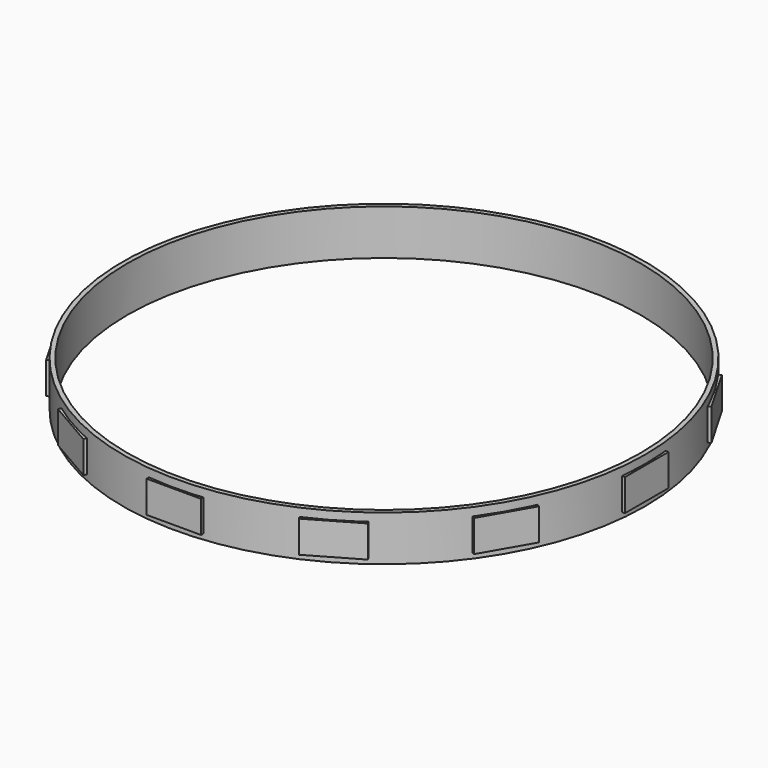
from build123d import *

# Parameters (mm, degrees)
F0_R     = 287.5
F0_R_2   = 282.5
F1_DEPTH = 50
F5_W     = 60
F5_H     = 35
F6_DEPTH = 2
F7_COUNT = 12


# Not quite as in the source:
# - the program builds the solid bodies; features that only make, move or delete a surface that nothing else refers to are left out


with BuildPart() as f1:
    # F0 (on Top) → F1 (new body)
    with BuildSketch(Plane.XY):
        Circle(F0_R)
        Circle(F0_R_2, mode=Mode.SUBTRACT)
    extrude(amount=F1_DEPTH)


with BuildPart() as f6:
    # F5 (on offset) → F6 (new body, symmetric)
    with BuildSketch(Plane.XZ.offset(287.2)):
        with Locations((0, 23.5)):
            Rectangle(F5_W, F5_H)
    extrude(amount=F6_DEPTH, both=True)


with BuildPart() as f7_1:
    # F7: instance of F6
    add(f6.part.rotate(Axis((0, 0, 0), (0, 0, -1)), 1 * 360 / F7_COUNT))


with BuildPart() as f7_2:
    # F7: instance of F6
    add(f6.part.rotate(Axis((0, 0, 0), (0, 0, -1)), 2 * 360 / F7_COUNT))


with BuildPart() as f7_3:
    # F7: instance of F6
    add(f6.part.rotate(Axis((0, 0, 0), (0, 0, -1)), 3 * 360 / F7_COUNT))


with BuildPart() as f7_4:
    # F7: instance of F6
    add(f6.part.rotate(Axis((0, 0, 0), (0, 0, -1)), 4 * 360 / F7_COUNT))


with BuildPart() as f7_5:
    # F7: instance of F6
    add(f6.part.rotate(Axis((0, 0, 0), (0, 0, -1)), 5 * 360 / F7_COUNT))


with BuildPart() as f7_6:
    # F7: instance of F6
    add(f6.part.rotate(Axis((0, 0, 0), (0, 0, -1)), 6 * 360 / F7_COUNT))


with BuildPart() as f7_7:
    # F7: instance of F6
    add(f6.part.rotate(Axis((0, 0, 0), (0, 0, -1)), 7 * 360 / F7_COUNT))


with BuildPart() as f7_8:
    # F7: instance of F6
    add(f6.part.rotate(Axis((0, 0, 0), (0, 0, -1)), 8 * 360 / F7_COUNT))


with BuildPart() as f7_9:
    # F7: instance of F6
    add(f6.part.rotate(Axis((0, 0, 0), (0, 0, -1)), 9 * 360 / F7_COUNT))


with BuildPart() as f7_10:
    # F7: instance of F6
    add(f6.part.rotate(Axis((0, 0, 0), (0, 0, -1)), 10 * 360 / F7_COUNT))


with BuildPart() as f7_11:
    # F7: instance of F6
    add(f6.part.rotate(Axis((0, 0, 0), (0, 0, -1)), 11 * 360 / F7_COUNT))


solid = Compound([f1.part, f6.part, f7_1.part, f7_2.part, f7_3.part, f7_4.part, f7_5.part, f7_6.part, f7_7.part, f7_8.part, f7_9.part, f7_10.part, f7_11.part])
